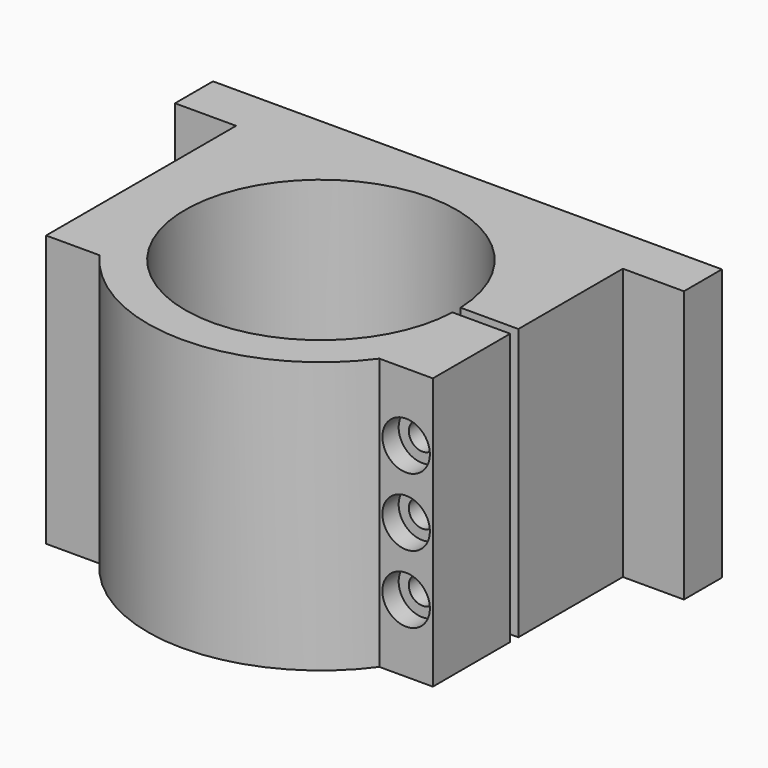
from build123d import *

# Parameters (mm, degrees)
F1_DEPTH       = 80
F3_D           = 8
F3_DEPTH       = 55
F3_CBORE_D     = 14
F3_CBORE_DEPTH = 6
F3_TIP         = 2.4034424761


# Not quite as in the source:
# - a feature of the source that left no trace in its solid (it failed there, or was rolled back) is left out


with BuildPart() as f1:
    # F0 (on Top) → F1 (new body)
    with BuildSketch(Plane.XY):
        with BuildLine():
            ThreePointArc((-31.6385840391, -14), (0, -3), (31.6385840391, -14))
            Line((31.6385840391, -14), (57, -14))
            Line((57, -14), (75, -14))
            Line((75, -14), (75, 0))
            Line((75, 0), (-75, 0))
            Line((-75, 0), (-75, -14))
            Line((-75, -14), (-57, -14))
            Line((-57, -14), (-31.6385840391, -14))
        make_face()
        with BuildLine():
            ThreePointArc((-41.2431812546, -84), (-50.5266061405, -47.0673185622), (-31.6385840391, -14))
            Line((-31.6385840391, -14), (-57, -14))
            Line((-57, -14), (-57, -84))
            Line((-57, -84), (-41.2431812546, -84))
        make_face()
        with BuildLine():
            ThreePointArc((0, -14), (27.748873851, -25.1902794182), (39.9718651053, -52.5))
            Line((39.9718651053, -52.5), (50.9779364039, -52.5))
            ThreePointArc((50.9779364039, -52.5), (45.5734008225, -31.1075309878), (31.6385840391, -14))
            Line((31.6385840391, -14), (0, -14))
        make_face()
        with BuildLine():
            ThreePointArc((-26.4575131106, -84), (-37.4165738677, -39.8578643763), (0, -14))
            Line((0, -14), (-31.6385840391, -14))
            ThreePointArc((-31.6385840391, -14), (-50.5266061405, -47.0673185622), (-41.2431812546, -84))
            Line((-41.2431812546, -84), (-26.4575131106, -84))
        make_face()
        with BuildLine():
            Line((57, -55.5), (50.9779364039, -55.5))
            ThreePointArc((50.9779364039, -55.5), (48.2622640947, -70.4849587338), (41.2431812546, -84))
            Line((41.2431812546, -84), (57, -84))
            Line((57, -84), (57, -55.5))
        make_face()
        with BuildLine():
            ThreePointArc((31.6385840391, -14), (45.5734008225, -31.1075309878), (50.9779364039, -52.5))
            Line((50.9779364039, -52.5), (57, -52.5))
            Line((57, -52.5), (57, -14))
            Line((57, -14), (31.6385840391, -14))
        make_face()
        with BuildLine():
            Line((41.2431812546, -84), (26.4575131106, -84))
            ThreePointArc((26.4575131106, -84), (0, -94), (-26.4575131106, -84))
            Line((-26.4575131106, -84), (-41.2431812546, -84))
            ThreePointArc((-41.2431812546, -84), (0, -105), (41.2431812546, -84))
        make_face()
        with BuildLine():
            Line((50.9779364039, -55.5), (39.9718651053, -55.5))
            ThreePointArc((39.9718651053, -55.5), (36.1424690986, -71.1383175213), (26.4575131106, -84))
            Line((26.4575131106, -84), (41.2431812546, -84))
            ThreePointArc((41.2431812546, -84), (48.2622640947, -70.4849587338), (50.9779364039, -55.5))
        make_face()
        with BuildLine():
            Line((-31.6385840391, -14), (0, -14))
            Line((0, -14), (31.6385840391, -14))
            ThreePointArc((31.6385840391, -14), (0, -3), (-31.6385840391, -14))
        make_face()
    extrude(amount=F1_DEPTH)

    # F3
    with Locations(Plane.XZ.offset(84)):
        with Locations((49.1215906273, 20), (49.1215906273, 40), (49.1215906273, 60)):
            CounterBoreHole(F3_D / 2, F3_CBORE_D / 2, F3_CBORE_DEPTH, depth=F3_DEPTH)
            with Locations((0, 0, -(F3_DEPTH + F3_TIP / 2))):  # 118° drill point
                Cone(0, F3_D / 2, F3_TIP, mode=Mode.SUBTRACT)


solid = f1.part
